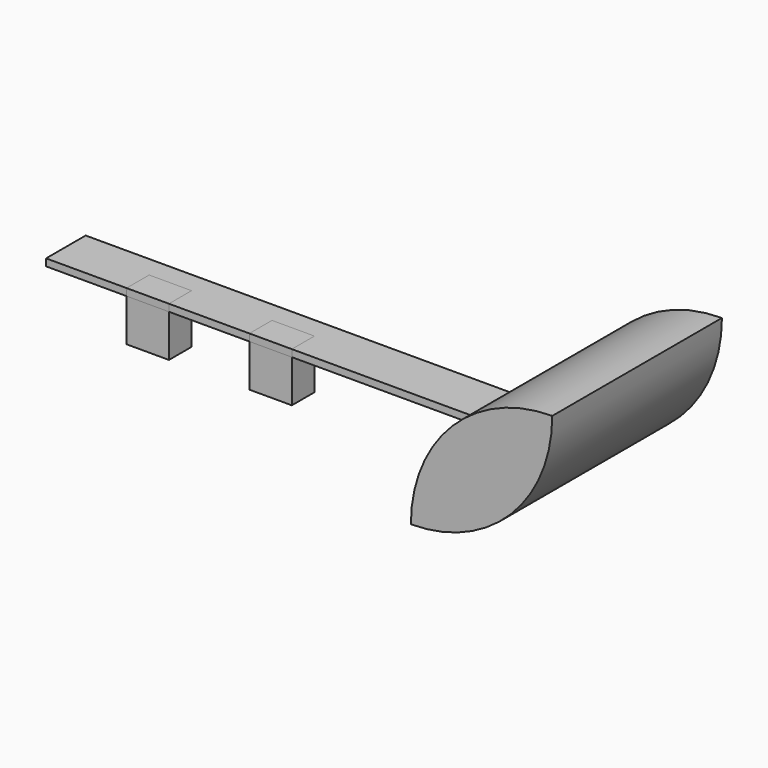
from build123d import *

# Parameters (mm, degrees)
F1_DEPTH = 1.27
F0_W     = 7.62
F0_H     = 5.08
F2_DEPTH = 7.62
F3_DEPTH = 1.27
F4_DEPTH = 25.4
F5_R     = 25.39999
F6_R     = 25.39999


# Not quite as in the source:
# - a fillet or chamfer is up to 0.001 mm smaller than in the source, because OpenCascade refuses the exact size


with BuildPart() as f1:
    # F0 (on Top) → F1 (new body)
    with BuildSketch(Plane.XY):
        Polygon((-56.5321096511, 32.319452062), (-145.4321096511, 32.319452062), (-145.4321096511, 23.429452062), (-130.9795096511, 23.429452062), (-130.9795096511, 28.509452062), (-123.3595096511, 28.509452062), (-123.3595096511, 23.429452062), (-108.9069096511, 23.429452062), (-108.9069096511, 28.509452062), (-101.2869096511, 28.509452062), (-101.2869096511, 23.429452062), (-56.5321096511, 23.429452062), align=None)
    extrude(amount=F1_DEPTH)

    # F0 (on Top) → F4 (join)
    with BuildSketch(Plane.XY):
        Polygon((-31.1321096511, 32.319452062), (-56.5321096511, 32.319452062), (-56.5321096511, 23.429452062), (-56.5321096511, -5.780547938), (-31.1321096511, -5.780547938), align=None)
    extrude(amount=F4_DEPTH)

    # F5 (radius 25.4 in the source; OpenCascade refuses exactly that, so slightly less here)
    f5_edges = [f1.edges().sort_by_distance(p)[0] for p in [
        (-31.13211, 13.269452, 0),
    ]]
    fillet(f5_edges, radius=F5_R)

    # F6 (radius 25.4 in the source; OpenCascade refuses exactly that, so slightly less here)
    f6_edges = [f1.edges().sort_by_distance(p)[0] for p in [
        (-56.53211, 13.269452, 25.4),
    ]]
    fillet(f6_edges, radius=F6_R)


with BuildPart() as f2:
    # F0 (on Top) → F2 (new body)
    with BuildSketch(Plane.XY):
        with Locations((-127.1695096511, 25.969452062)):
            Rectangle(F0_W, F0_H)
    extrude(amount=-F2_DEPTH)


with BuildPart() as f2b:
    # F0 (on Top) → F2, piece 2 (new body)
    with BuildSketch(Plane.XY):
        with Locations((-105.0969096511, 25.969452062)):
            Rectangle(F0_W, F0_H)
    extrude(amount=-F2_DEPTH)


with BuildPart() as f3:
    # F0 (on Top) → F3 (new body)
    with BuildSketch(Plane.XY):
        with Locations((-127.1695096511, 25.969452062)):
            Rectangle(F0_W, F0_H)
    extrude(amount=F3_DEPTH)


with BuildPart() as f3b:
    # F0 (on Top) → F3, piece 2 (new body)
    with BuildSketch(Plane.XY):
        with Locations((-105.0969096511, 25.969452062)):
            Rectangle(F0_W, F0_H)
    extrude(amount=F3_DEPTH)


solid = Compound([f1.part, f2.part, f2b.part, f3.part, f3b.part])
